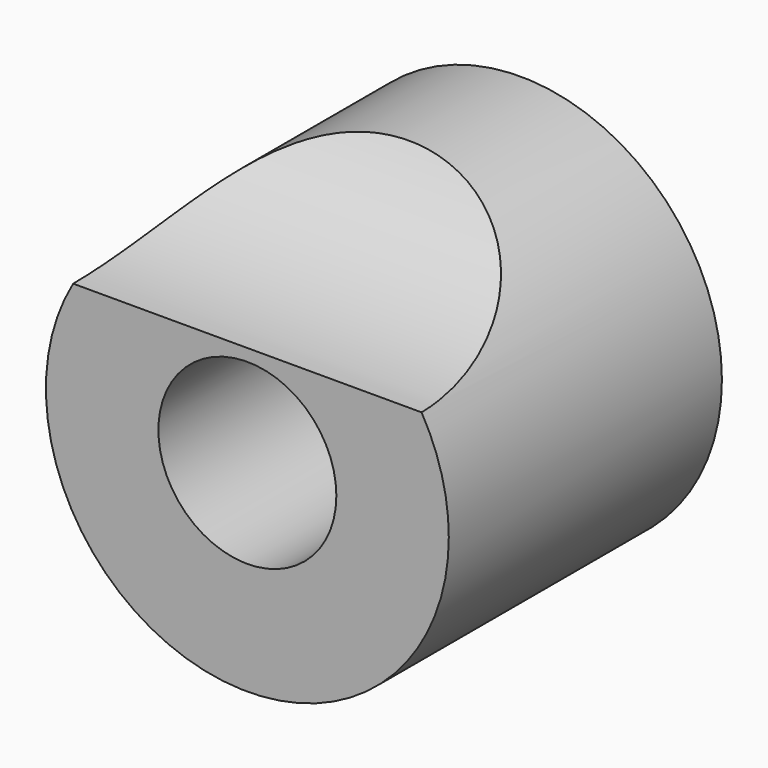
from build123d import *

# Parameters (mm, degrees)
F0_R     = 12.45
F0_R_2   = 5.5
F1_DEPTH = 21.1
F3_DEPTH = 12.5


with BuildPart() as f1:
    # F0 (on Front) → F1 (new body)
    with BuildSketch(Plane.XZ):
        Circle(F0_R)
        Circle(F0_R_2, mode=Mode.SUBTRACT)
    extrude(amount=F1_DEPTH)

    # F2 (on Right) → F3 (cut, symmetric)
    with BuildSketch(Plane.YZ):
        with BuildLine():
            Line((-8.6, 12.45), (-21.1, 12.45))
            Line((-21.1, 12.45), (-21.1, 6.25))
            ThreePointArc((-21.1, 6.25), (-14.1385472549, 7.9156194655), (-8.6, 12.45))
        make_face()
    extrude(amount=F3_DEPTH, both=True, mode=Mode.SUBTRACT)


solid = f1.part
